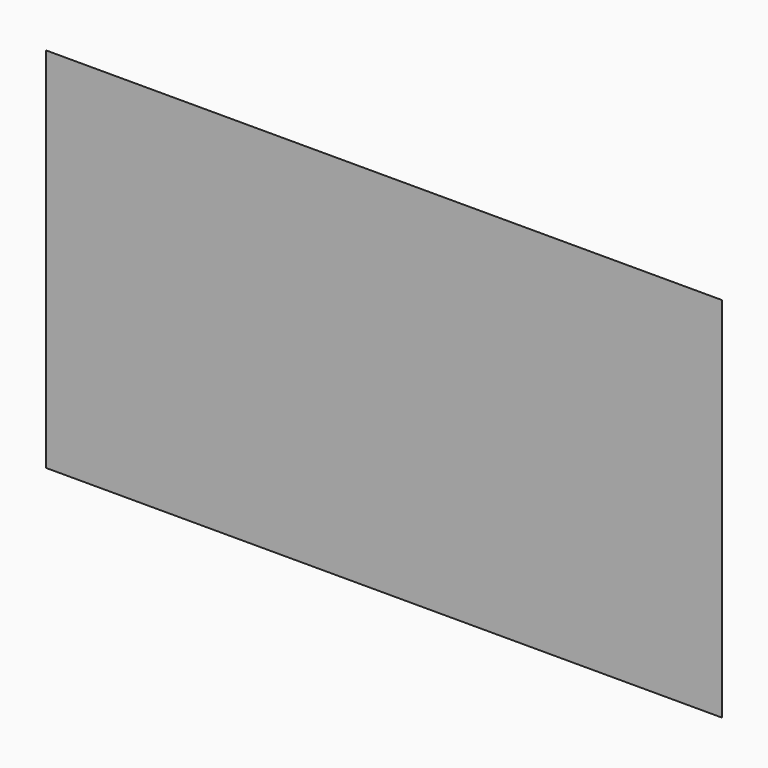
from build123d import *

# Parameters (mm, degrees)
F0_W        = 56.1207598075
F0_H        = 32.6107107103
F1_DEPTH    = 2.794
F2_T1_DEPTH = 82.2490589653
F2_T3_DEPTH = 58.739009868


# Not quite as in the source:
# - a fillet or chamfer that OpenCascade refuses, or shapes differently, is made with other operations: its cross-section is extruded or revolved along the edge and cut away or added


with BuildPart() as f1:
    # F0 (on Front) → F1 (new body)
    with BuildSketch(Plane.XZ):
        with Locations((-31.2835318036, 16.3053553551)):
            Rectangle(F0_W, F0_H)
    extrude(amount=F1_DEPTH)

    # F2: chamfer of 5.08 on 4 edges, made by hand

    # F2_s2 → F2_t1 (cut)
    with BuildSketch(Plane.YZ.offset(-72.4080612863)):
        Polygon((-5.08, 32.6107107103), (0, 27.5307107103), (0, 32.6107107103), align=None)
        Polygon((-5.08, 0), (0, 5.08), (0, 0), align=None)
    extrude(amount=F2_T1_DEPTH, mode=Mode.SUBTRACT)

    # F2_s4 → F2_t3 (cut)
    with BuildSketch(Plane.XY.offset(-13.0641495789)):
        Polygon((-3.2231518999, -5.08), (-8.3031518999, 0), (-3.2231518999, 0), align=None)
        Polygon((-59.3439117074, -5.08), (-54.2639117074, 0), (-59.3439117074, 0), align=None)
    extrude(amount=F2_T3_DEPTH, mode=Mode.SUBTRACT)


solid = f1.part
